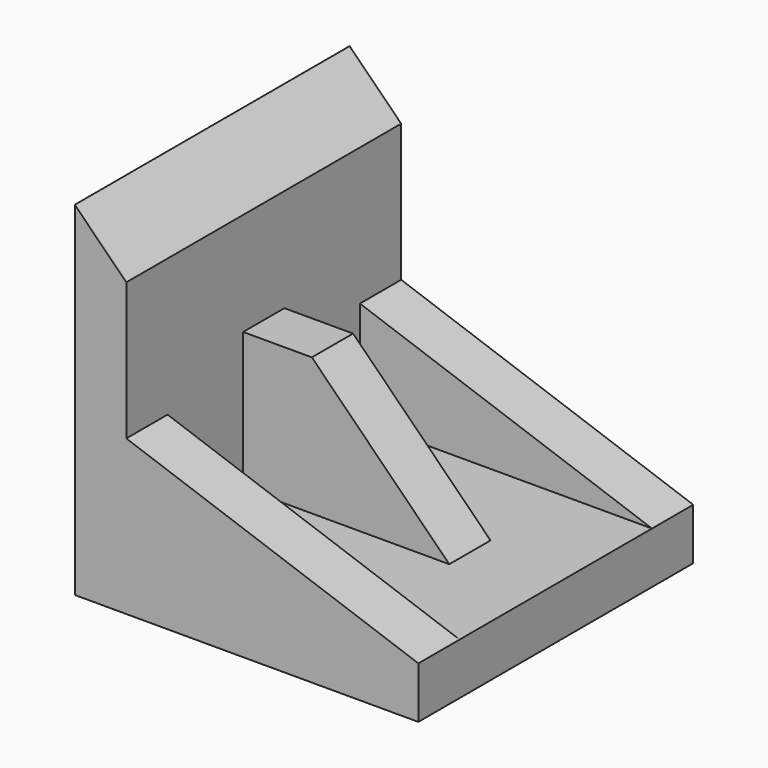
from build123d import *

# Parameters (mm, degrees)
F1_DEPTH = 127
F3_DEPTH = 38.1
F4_DEPTH = 19.05


# Not quite as in the source:
# - a pattern or mirror of a feature is missing from the dataset's text; its kind, count and spacing are read off the source's solid


with BuildPart() as f1:
    # F0 (on Front) → F1 (new body, symmetric)
    with BuildSketch(Plane.XZ):
        Polygon((0, 254), (0, 0), (254, 0), (254, 38.1), (190.5, 38.1), (38.1, 38.1), (38.1, 139.7), (38.1, 215.9), align=None)
    extrude(amount=F1_DEPTH, both=True)

    # F2 (on face) → F3 (join)
    with BuildSketch(Plane.XZ.offset(127)):
        Polygon((254, 38.1), (38.1, 114.3), (38.1, 38.1), align=None)
    f3 = extrude(amount=-F3_DEPTH)

    # F3_copies: F3 across plane
    add(f3.mirror(Plane.ZX))

    # F0 (on Front) → F4 (join, symmetric)
    with BuildSketch(Plane.XZ):
        Polygon((0, 254), (0, 0), (254, 0), (254, 38.1), (190.5, 38.1), (38.1, 38.1), (38.1, 139.7), (38.1, 215.9), align=None)
        Polygon((38.1, 38.1), (190.5, 38.1), (88.9, 139.7), (38.1, 139.7), align=None)
    extrude(amount=F4_DEPTH, both=True)


solid = f1.part
